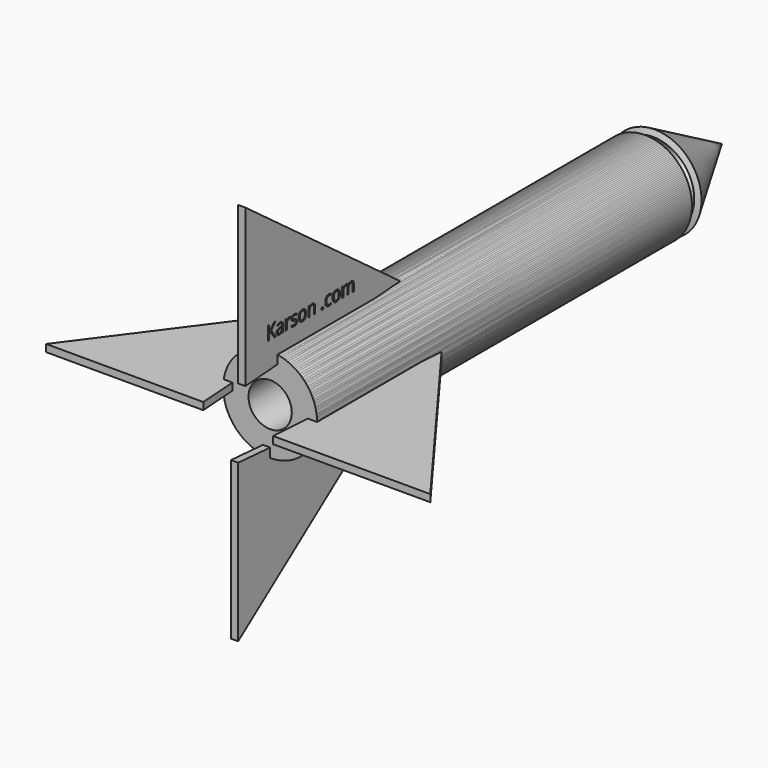
from build123d import *

# Parameters (mm, degrees)
F3_DEPTH     = 3
F4_COUNT     = 4
F5_R         = 9
F6_DEPTH     = 64
F7_TEXT_SIZE = 7.9317716882
F8_DEPTH     = 1


# Not quite as in the source:
# - Text() gives the source's letters only with a copy of the font that has no kerning and outlines rounded to 1/6400 em; it was checked with that copy


with BuildPart() as f1:
    # F0 (on Top) → F1 (revolve)
    with BuildSketch(Plane.XY):
        Polygon((19.1731275601, 77.6207819581), (0, 111.9795814157), (0, 106.3221991062), (16.3165574432, 77.6207819581), align=None)
        Polygon((19.5263698697, 76.9877615165), (19.1731275601, 77.6207819581), (16.3165574432, 77.6207819581), (17.1338901608, 76.183064023), align=None)
    revolve(axis=Axis((0, -5.4250992835, 0), (0, -1, 0)))


with BuildPart() as f1b:
    # F0 (on Top) → F1, piece 2 (revolve)
    with BuildSketch(Plane.XY):
        Polygon((10.1160742342, 71.9746053219), (0, 71.9746053219), (0, -122.8297799826), (19.5263698697, -122.8297799826), (19.5263698697, 71.9746053219), (15.7622490078, 71.9746053219), (10.1160742342, 77.6207819581), align=None)
    revolve(axis=Axis((0, -5.4250992835, 0), (0, -1, 0)))

    # F2 (on Top) → F3 (join)
    with BuildSketch(Plane.XY):
        Polygon((-14.5053261418, -139.4455954432), (-20.2234701277, -58.9680090296), (-79.8727588557, -139.4455954432), align=None)
    extrude(amount=F3_DEPTH)


with BuildPart() as f4_1:
    # F4: instance of F1b
    add(f1b.part.rotate(Axis((0, -122.8297799826, 0), (0, 1, 0)), 1 * 360 / F4_COUNT))


with BuildPart() as f4_2:
    # F4: instance of F1b
    add(f1b.part.rotate(Axis((0, -122.8297799826, 0), (0, 1, 0)), 2 * 360 / F4_COUNT))


with BuildPart() as f4_3:
    # F4: instance of F1b
    add(f1b.part.rotate(Axis((0, -122.8297799826, 0), (0, 1, 0)), 3 * 360 / F4_COUNT))


with BuildPart() as f6_tool:
    # F5 (on face) → F6 (new body)
    with BuildSketch(Plane.XZ.offset(122.8297799826)):
        Circle(F5_R)
    extrude(amount=-F6_DEPTH)


with BuildPart() as f1b_1:
    add(f1b.part)

    # F6: cut by f6_tool
    add(f6_tool.part, mode=Mode.SUBTRACT)


with BuildPart() as f4_1_1:
    add(f4_1.part)

    # F6: cut by f6_tool
    add(f6_tool.part, mode=Mode.SUBTRACT)

    # F7 (on face) → F8 (cut)
    with BuildSketch(Plane.YZ.offset(3)):
        with Locations((-128.5095512867, 26.2271761894)):
            Text('Karson .com', F7_TEXT_SIZE, font='Open Sans', text_align=(TextAlign.LEFT, TextAlign.BOTTOM))
    extrude(amount=-F8_DEPTH, mode=Mode.SUBTRACT)


with BuildPart() as f4_2_1:
    add(f4_2.part)

    # F6: cut by f6_tool
    add(f6_tool.part, mode=Mode.SUBTRACT)


with BuildPart() as f4_3_1:
    add(f4_3.part)

    # F6: cut by f6_tool
    add(f6_tool.part, mode=Mode.SUBTRACT)


solid = Compound([f1.part, f1b_1.part, f4_1_1.part, f4_2_1.part, f4_3_1.part])
